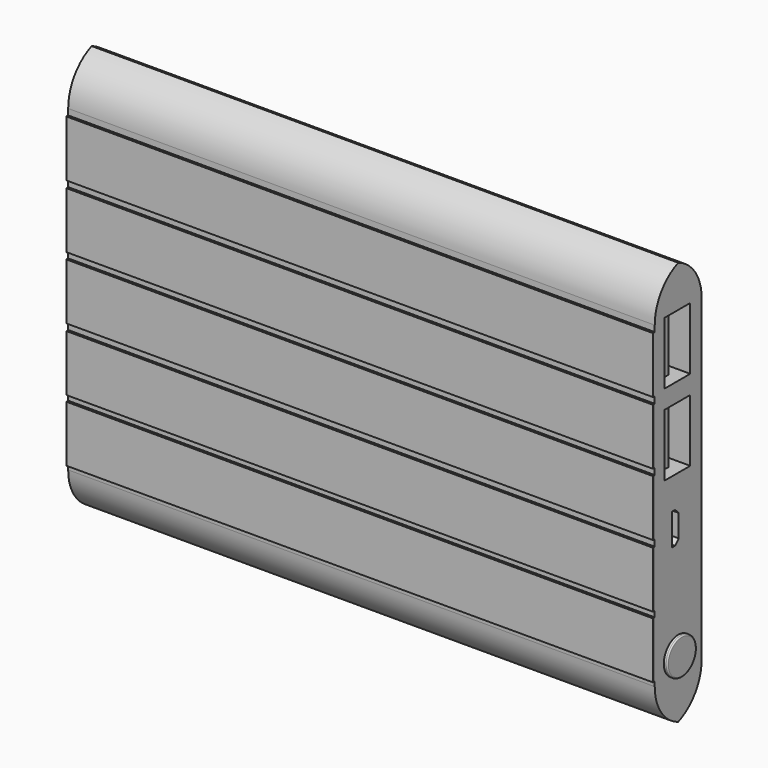
from build123d import *

# Parameters (mm, degrees)
F0_W        = 127
F0_H        = 88.9
F1_DEPTH    = 12.7
F2_T1_DEPTH = 177
F3_W        = 1.8
F3_H        = 6.85
F4_DEPTH    = 16.4
F3_W_2      = 7
F3_H_2      = 13.5
F3_W_3      = 2.7532497272
F3_H_3      = 12.2928316705
F5_DEPTH    = 16.4
F6_SIZE     = 1
F7_DEPTH    = 2.794
F8_DEPTH    = 1.8542
F3_R        = 3.9463270772
F9_DEPTH    = 0.762
F10_R       = 0.254
F13_W       = 127
F13_H       = 12.192
F14_DEPTH   = 0.5
F15_R       = 3.9211509086
F16_DEPTH   = 1.27


# Not quite as in the source:
# - a fillet or chamfer that OpenCascade refuses, or shapes differently, is made with other operations: its cross-section is extruded or revolved along the edge and cut away or added
# - the program builds the solid bodies; features that only make, move or delete a surface that nothing else refers to are left out


with BuildPart() as f1:
    # F0 (on Front) → F1 (new body)
    with BuildSketch(Plane.XZ):
        Rectangle(F0_W, F0_H)
    extrude(amount=F1_DEPTH)

    # F2: fillet of radius 10 on 4 edges, made by hand

    # F2_s2 → F2_t1 (cut)
    with BuildSketch(Plane.YZ.offset(-88.5)):
        with BuildLine():
            ThreePointArc((-2.7, 44.45), (-9.7710678119, 41.5210678119), (-12.7, 34.45))
            Line((-12.7, 34.45), (-12.7, 44.45))
            Line((-12.7, 44.45), (-2.7, 44.45))
        make_face()
        with BuildLine():
            ThreePointArc((-10, 44.45), (-2.9289321881, 41.5210678119), (0, 34.45))
            Line((0, 34.45), (0, 44.45))
            Line((0, 44.45), (-10, 44.45))
        make_face()
        with BuildLine():
            ThreePointArc((-2.7, -44.45), (-9.7710678119, -41.5210678119), (-12.7, -34.45))
            Line((-12.7, -34.45), (-12.7, -44.45))
            Line((-12.7, -44.45), (-2.7, -44.45))
        make_face()
        with BuildLine():
            ThreePointArc((-10, -44.45), (-2.9289321881, -41.5210678119), (0, -34.45))
            Line((0, -34.45), (0, -44.45))
            Line((0, -44.45), (-10, -44.45))
        make_face()
    extrude(amount=F2_T1_DEPTH, mode=Mode.SUBTRACT)

    # F3 (on face) → F4 (cut)
    with BuildSketch(Plane.YZ.offset(63.5)):
        with Locations((-7.1068273082, -6.4043554038)):
            Rectangle(F3_W, F3_H)
    extrude(amount=-F4_DEPTH, mode=Mode.SUBTRACT)

    # F3 (on face) → F5 (cut)
    with BuildSketch(Plane.YZ.offset(63.5)):
        with Locations((-6.591425851, 10.4809925538)):
            Rectangle(F3_W_2, F3_H_2)
        with Locations((-7.9680507146, 10.4750713799)):
            Rectangle(F3_W_3, F3_H_3, mode=Mode.SUBTRACT)
        with Locations((-6.591425851, 28.0195952505)):
            Rectangle(F3_W_2, F3_H_2)
        with Locations((-7.9680507146, 28.0764119234)):
            Rectangle(F3_W_3, F3_H_3, mode=Mode.SUBTRACT)
    extrude(amount=-F5_DEPTH, mode=Mode.SUBTRACT)

    # F6
    f6_edges = [f1.edges().sort_by_distance(p)[0] for p in [
        (55.3, -6.206827, -2.979355),
        (55.3, -6.206827, -9.829355),
    ]]
    chamfer(f6_edges, length=F6_SIZE)

    # F7 (add): faces of the model
    f7_faces = [f1.faces().sort_by_distance(p)[0] for p in [
        (63.5, -7.9680507146, 10.4750713799),
        (63.5, -7.9680507146, 28.0764119234),
    ]]
    extrude(f7_faces, amount=-F7_DEPTH)

    # F8 (cut): faces of the model
    f8_faces = [f1.faces().sort_by_distance(p)[0] for p in [
        (63.5, -7.9680507146, 10.4750713799),
        (63.5, -7.9680507146, 28.0764119234),
    ]]
    extrude(f8_faces, amount=-F8_DEPTH, mode=Mode.SUBTRACT)

    # F3 (on face) → F9 (join)
    with BuildSketch(Plane.YZ.offset(63.5)):
        with Locations((-6.3012135215, -31.0900993645)):
            Circle(F3_R)
    extrude(amount=F9_DEPTH)

    # F10
    f10_edges = [f1.edges().sort_by_distance(p)[0] for p in [
        (64.262, -10.247541, -31.090099),
    ]]
    fillet(f10_edges, radius=F10_R)

    # F13 (on face) → F14 (join)
    with BuildSketch(Plane.XZ.offset(12.7)):
        with Locations((0, 27.0355174699)):
            Rectangle(F13_W, F13_H)
        with Locations((-2.0266e-06, 13.3711864791)):
            Rectangle(F13_W, F13_H)
        with Locations((-2.0266e-06, -0.2175037199)):
            Rectangle(F13_W, F13_H)
        with Locations((-2.0266e-06, -13.8689222195)):
            Rectangle(F13_W, F13_H)
        with Locations((-2.0266e-06, -27.337996141)):
            Rectangle(F13_W, F13_H)
    extrude(amount=F14_DEPTH)

    # F15 (on face) → F16 (cut)
    with BuildSketch(Plane(origin=(-63.5, 0, 0), x_dir=(0, -1, 0), z_dir=(-1, 0, 0))):
        with Locations((7.0751463063, -30.106594786)):
            Circle(F15_R)
        with Locations((7.0751463063, 29.6837498702)):
            Circle(F15_R)
    extrude(amount=-F16_DEPTH, mode=Mode.SUBTRACT)

    # F17: fillet of radius 2.54 on 2 edges, made by hand

    # F17_s1 → F17_t2 (revolve)
    with BuildSketch(Plane.XY.offset(-30.106594786)):
        with BuildLine():
            ThreePointArc((-63.5, -10.9962972149), (-62.5702954744, -10.0665926893), (-62.23, -8.7965926893))
            Line((-62.23, -8.7965926893), (-62.23, -10.9962972149))
            Line((-62.23, -10.9962972149), (-63.5, -10.9962972149))
        make_face()
    revolve(axis=Axis((-62.23, -7.0751463063, -30.106594786), (-1, 0, 0)))

    # F17_s3 → F17_t4 (revolve)
    with BuildSketch(Plane.XY.offset(29.6837498702)):
        with BuildLine():
            ThreePointArc((-63.5, -10.9962972149), (-62.5702954744, -10.0665926893), (-62.23, -8.7965926893))
            Line((-62.23, -8.7965926893), (-62.23, -10.9962972149))
            Line((-62.23, -10.9962972149), (-63.5, -10.9962972149))
        make_face()
    revolve(axis=Axis((-62.23, -7.0751463063, 29.6837498702), (-1, 0, 0)))


solid = f1.part
